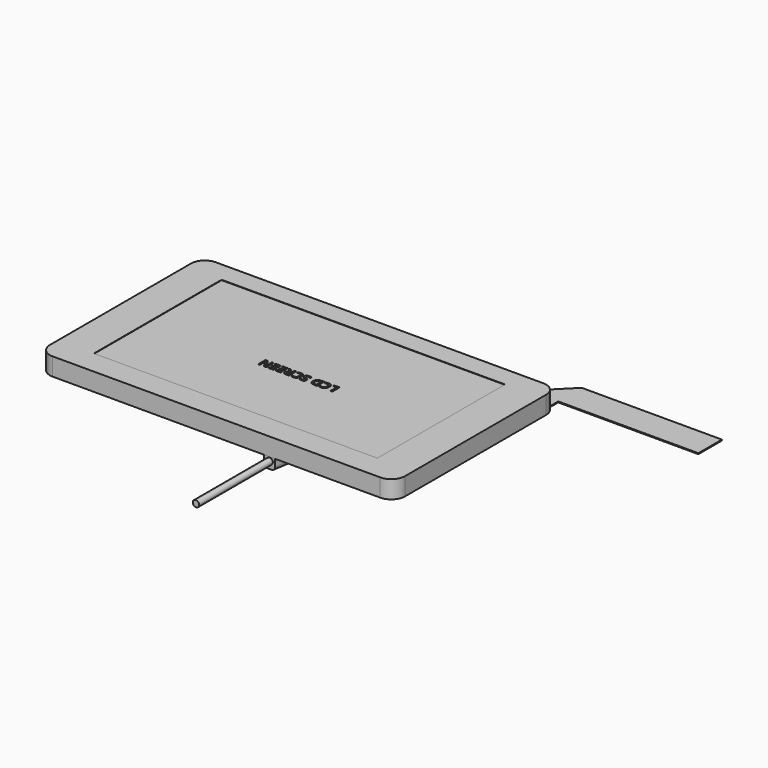
from build123d import *

# Parameters (mm, degrees)
F0_W          = 192.96
F0_H          = 110.76
F0_R          = 1.5
F0_W_2        = 67
F0_H_2        = 78.27
F0_W_3        = 45
F0_H_3        = 4
F1_DEPTH      = 9.7
F2_R          = 7.5
F3_W          = 154
F3_H          = 86.72
F4_DEPTH      = 0.2
F5_DEPTH      = 3.3
F6_W          = 65
F6_H          = 56
F7_DEPTH      = 0.8
F8_R          = 3
F9_W          = 6
F9_H          = 21
F10_DEPTH     = 2.8
F9_W_2        = 7.5
F9_H_2        = 4.2
F9_H_3        = 1.5
F11_DEPTH     = 3
F9_W_3        = 12
F9_H_4        = 13
F9_W_4        = 2
F12_DEPTH     = 6.8
F13_R         = 1
F14_DEPTH     = 3
F15_DEPTH     = 5
F16_R         = 6.0597839978
F17_DEPTH     = 1
F19_DEPTH     = 0.5
F20_TEXT_SIZE = 6.9444444444
F21_DEPTH     = 1
F25_DEPTH     = 3.8
F26_R         = 2
F28_DEPTH     = 50
F29_W         = 6.1920173466
F29_H         = 2.4811383337
F30_DEPTH     = 8


# Not quite as in the source:
# - Text() gives the source's letters only with a copy of the font that has no kerning and outlines rounded to 1/6400 em; it was checked with that copy


with BuildPart() as f1:
    # F0 (on Top) → F1 (new body)
    with BuildSketch(Plane.XY):
        Rectangle(F0_W, F0_H)
        Polygon((-77, 44.37), (77, 44.37), (77, -42.35), (39.98, -42.35), (39.98, -49.08), (17.98, -49.08), (17.98, -53.08), (-27.02, -53.08), (-27.02, -49.08), (-27.02, -42.35), (-77, -42.35), align=None, mode=Mode.SUBTRACT)
        Polygon((77, -42.35), (77, 44.37), (-77, 44.37), (-77, -42.35), (-27.02, -42.35), (-27.02, 35.92), (39.98, 35.92), (39.98, -42.35), align=None)
        with Locations((-63.1, -31.85)):
            Circle(F0_R, mode=Mode.SUBTRACT)
        with Locations((63.1, -31.85)):
            Circle(F0_R, mode=Mode.SUBTRACT)
        with Locations((-63.1, 33.8)):
            Circle(F0_R, mode=Mode.SUBTRACT)
        with Locations((63.1, 33.8)):
            Circle(F0_R, mode=Mode.SUBTRACT)
        with Locations((6.48, -3.215)):
            Rectangle(F0_W_2, F0_H_2)
        with Locations((-4.52, -51.08)):
            Rectangle(F0_W_3, F0_H_3)
        Polygon((39.98, -49.08), (39.98, -42.35), (-27.02, -42.35), (-27.02, -49.08), (17.98, -49.08), align=None)
        with Locations((63.1, 33.8)):
            Circle(F0_R)
        with Locations((63.1, -31.85)):
            Circle(F0_R)
        with Locations((-63.1, -31.85)):
            Circle(F0_R)
        with Locations((-63.1, 33.8)):
            Circle(F0_R)
    extrude(amount=F1_DEPTH)

    # F2
    f2_edges = [f1.edges().sort_by_distance(p)[0] for p in [
        (-96.48, -55.38, 4.85),
        (96.48, -55.38, 4.85),
        (96.48, 55.38, 4.85),
        (-96.48, 55.38, 4.85),
    ]]
    fillet(f2_edges, radius=F2_R)

    # F3 (on face) → F4 (cut)
    with BuildSketch(Plane.XY.offset(9.7)):
        with Locations((0, 1.01)):
            Rectangle(F3_W, F3_H)
    extrude(amount=-F4_DEPTH, mode=Mode.SUBTRACT)

    # F0 (on Top) → F5 (cut)
    with BuildSketch(Plane.XY):
        with Locations((6.48, -3.215)):
            Rectangle(F0_W_2, F0_H_2)
        Polygon((39.98, -49.08), (39.98, -42.35), (-27.02, -42.35), (-27.02, -49.08), (17.98, -49.08), align=None)
        with Locations((-4.52, -51.08)):
            Rectangle(F0_W_3, F0_H_3)
    extrude(amount=F5_DEPTH, mode=Mode.SUBTRACT)

    # F0 (on Top) → F15 (cut)
    with BuildSketch(Plane.XY):
        with Locations((63.1, 33.8)):
            Circle(F0_R)
        with Locations((63.1, -31.85)):
            Circle(F0_R)
        with Locations((-63.1, 33.8)):
            Circle(F0_R)
        with Locations((-63.1, -31.85)):
            Circle(F0_R)
    extrude(amount=F15_DEPTH, mode=Mode.SUBTRACT)

    # F20 (on face) → F21 (cut)
    with BuildSketch(Plane.XY.offset(9.5)):
        with Locations(Location((24.2769248473, -1.2744037575), (0, 0, -180))):
            Text('LCD SCREEN', F20_TEXT_SIZE, font='Open Sans', font_style=FontStyle.BOLD, text_align=(TextAlign.LEFT, TextAlign.BOTTOM))
    extrude(amount=-F21_DEPTH, mode=Mode.SUBTRACT)


with BuildPart() as f7:
    # F6 (on Top) → F7 (new body, symmetric)
    with BuildSketch(Plane.XY):
        with Locations((6.48, 4.42)):
            Rectangle(F6_W, F6_H)
    extrude(amount=F7_DEPTH, both=True)

    # F8
    f8_edges = [f7.edges().sort_by_distance(p)[0] for p in [
        (38.98, -23.58, 0),
        (-26.02, -23.58, 0),
        (-26.02, 32.42, 0),
        (38.98, 32.42, 0),
    ]]
    fillet(f8_edges, radius=F8_R)

    # F9 (on face) → F10 (join)
    with BuildSketch(Plane(origin=(0, 0, -0.8), x_dir=(1, 0, 0), z_dir=(0, 0, -1))):
        with Locations((35.98, -6.5)):
            Rectangle(F9_W, F9_H)
    extrude(amount=F10_DEPTH)

    # F9 (on face) → F11 (join)
    with BuildSketch(Plane(origin=(0, 0, -0.8), x_dir=(1, 0, 0), z_dir=(0, 0, -1))):
        with Locations((28.63, 21.48)):
            Rectangle(F9_W_2, F9_H_2)
        with Locations((28.63, 24.33)):
            Rectangle(F9_W_2, F9_H_3)
    extrude(amount=F11_DEPTH)

    # F9 (on face) → F12 (join)
    with BuildSketch(Plane(origin=(0, 0, -0.8), x_dir=(1, 0, 0), z_dir=(0, 0, -1))):
        with Locations((-20.02, 9.78)):
            Rectangle(F9_W_3, F9_H_4)
        with Locations((-27.02, 9.78)):
            Rectangle(F9_W_4, F9_H_4)
    extrude(amount=F12_DEPTH)

    # F13 (on face) → F14 (cut)
    with BuildSketch(Plane(origin=(0, 0, -0.8), x_dir=(1, 0, 0), z_dir=(0, 0, -1))):
        with Locations((35.98, -29.42)):
            Circle(F13_R)
        with Locations((35.98, 20.58)):
            Circle(F13_R)
        with Locations((-23.02, 20.58)):
            Circle(F13_R)
        with Locations((-23.02, -29.42)):
            Circle(F13_R)
    extrude(amount=-F14_DEPTH, mode=Mode.SUBTRACT)

    # F16 (on face) → F17 (cut)
    with BuildSketch(Plane(origin=(0, 0, -0.8), x_dir=(1, 0, 0), z_dir=(0, 0, -1))):
        Circle(F16_R)
    extrude(amount=-F17_DEPTH, mode=Mode.SUBTRACT)


with BuildPart() as f19:
    # F18 (on face) → F19 (new body)
    with BuildSketch(Plane(origin=(0, 0, -3.6), x_dir=(1, 0, 0), z_dir=(0, 0, -1))):
        Polygon((38.98, 1.5), (38.98, -14.5), (72.98, -14.5), (72.98, -65.5), (88.98, -81.5), (165.1187316179, -81.5), (165.1187316179, -65.5), (88.98, -65.5), (88.98, -14.5), (72.98, 1.5), align=None)
    extrude(amount=-F19_DEPTH)


with BuildPart() as f25:
    # F24 (on plane+point) → F25 (new body, symmetric)
    with BuildSketch(Plane.XY.offset(-2.3)):
        Polygon((33.93, -40.08), (33.93, -28.08), (28.63, -28.08), (23.33, -28.08), (23.33, -40.08), (25.63, -55.08), (28.63, -55.08), (31.63, -55.08), align=None)
    extrude(amount=F25_DEPTH, both=True)

    # F26
    f26_edges = [f25.edges().sort_by_distance(p)[0] for p in [
        (24.48, -47.58, -6.1),
        (23.33, -34.08, -6.1),
        (24.48, -47.58, 1.5),
        (23.33, -34.08, 1.5),
        (32.78, -47.58, -6.1),
        (33.93, -34.08, -6.1),
        (33.93, -34.08, 1.5),
        (32.78, -47.58, 1.5),
    ]]
    fillet(f26_edges, radius=F26_R)

    # F27 (on face) → F28 (join)
    with BuildSketch(Plane.XZ.offset(55.08)):
        with BuildLine():
            ThreePointArc((30.38, -2.3), (28.63, -0.55), (26.88, -2.3))
            Line((26.88, -2.3), (30.38, -2.3))
        make_face()
        with BuildLine():
            Line((30.38, -2.3), (26.88, -2.3))
            ThreePointArc((26.88, -2.3), (28.63, -4.05), (30.38, -2.3))
        make_face()
    extrude(amount=F28_DEPTH)

    # F29 (on face) → F30 (join)
    with BuildSketch(Plane(origin=(0, -28.08, 0), x_dir=(-1, 0, 0), z_dir=(0, 1, 0))):
        with Locations((-28.63, -2.3)):
            Rectangle(F29_W, F29_H)
    extrude(amount=F30_DEPTH)


solid = Compound([f1.part, f7.part, f19.part, f25.part])
